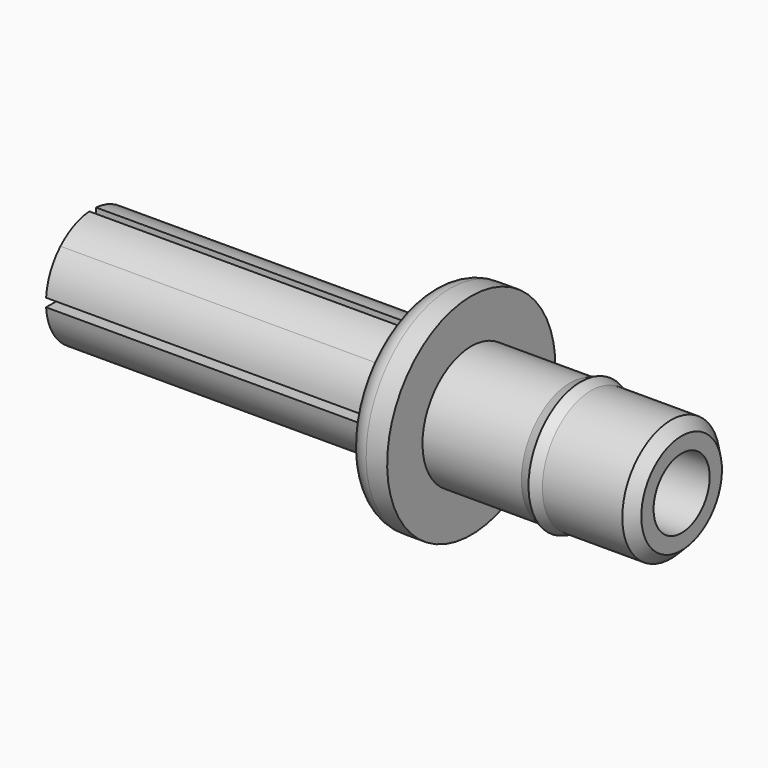
from build123d import *

# Parameters (mm, degrees)
F3_DEPTH = 15
F4_DEPTH = 15
F5_DEPTH = 15
F7_R     = 1


# Not quite as in the source:
# - after a boolean that leaves OpenCascade's solid faulty, fix() repairs it
# - a feature of the source that left no trace in its solid (it failed there, or was rolled back) is left out


with BuildPart() as f1:
    # F0 (on Front) → F1 (revolve)
    with BuildSketch(Plane.XZ):
        Polygon((2.7639019594, 2.7772041211), (2.7639019594, 1.666), (15.7639019594, 1.666), (15.7639019594, 2.3962433916), (15.2639019594, 2.9), (11.4639019594, 2.9), (10.9639019594, 3.1), (10.4639019594, 2.9), (5.7639019594, 2.9), (5.7639019594, 5), (3.7639019594, 5), (3.7639019594, 2.7772041211), align=None)
    revolve(axis=Axis((8.0730360566, 0, 0), (1, 0, 0)))

    # F2 (on face) → F3 (join)
    with BuildSketch(Plane(origin=(2.7639019594, 0, 0), x_dir=(0, -1, 0), z_dir=(-1, 0, 0))):
        with BuildLine():
            ThreePointArc((-1.1878670343, 1.1681300907), (-0.7352206258, 1.4949938566), (-0.2, 1.6539516317))
            Line((-0.2, 1.6539516317), (-0.2, 2.7699932726))
            ThreePointArc((-0.2, 2.7699932726), (-1.249471885, 2.4802586032), (-2.1069209339, 1.8093498579))
            ThreePointArc((-2.1069209339, 1.8093498579), (-2.5677957056, 1.0579640563), (-2.7699932726, 0.2))
            Line((-2.7699932726, 0.2), (-1.6539516317, 0.2))
            ThreePointArc((-1.6539516317, 0.2), (-1.5011003633, 0.7226712249), (-1.1878670343, 1.1681300907))
        make_face()
    extrude(amount=F3_DEPTH)

    # F2 (on face) → F4 (join)
    with BuildSketch(Plane(origin=(2.7639019594, 0, 0), x_dir=(0, -1, 0), z_dir=(-1, 0, 0))):
        with BuildLine():
            Line((0.2, 2.7699932726), (0.2, 1.6539516317))
            ThreePointArc((0.2, 1.6539516317), (0.75564146, 1.4847767455), (1.2194377654, 1.1351332681))
            ThreePointArc((1.2194377654, 1.1351332681), (1.5108640621, 0.7020297614), (1.6539516317, 0.2))
            Line((1.6539516317, 0.2), (2.7699932726, 0.2))
            ThreePointArc((2.7699932726, 0.2), (2.5121240066, 1.1841012226), (1.917164961, 2.0093136247))
            ThreePointArc((1.917164961, 2.0093136247), (1.1248356545, 2.5392139493), (0.2, 2.7699932726))
        make_face()
    extrude(amount=F4_DEPTH)

    # F2 (on face) → F5 (join)
    with BuildSketch(Plane(origin=(2.7639019594, 0, 0), x_dir=(0, -1, 0), z_dir=(-1, 0, 0))):
        with BuildLine():
            ThreePointArc((-1.1878670343, 1.1681300907), (-0.7352206258, 1.4949938566), (-0.2, 1.6539516317))
            Line((-0.2, 1.6539516317), (-0.2, 2.7699932726))
            ThreePointArc((-0.2, 2.7699932726), (-1.249471885, 2.4802586032), (-2.1069209339, 1.8093498579))
            ThreePointArc((-2.1069209339, 1.8093498579), (-2.5677957056, 1.0579640563), (-2.7699932726, 0.2))
            Line((-2.7699932726, 0.2), (-1.6539516317, 0.2))
            ThreePointArc((-1.6539516317, 0.2), (-1.5011003633, 0.7226712249), (-1.1878670343, 1.1681300907))
        make_face()
        with BuildLine():
            Line((0.2, 2.7699932726), (0.2, 1.6539516317))
            ThreePointArc((0.2, 1.6539516317), (0.75564146, 1.4847767455), (1.2194377654, 1.1351332681))
            ThreePointArc((1.2194377654, 1.1351332681), (1.5108640621, 0.7020297614), (1.6539516317, 0.2))
            Line((1.6539516317, 0.2), (2.7699932726, 0.2))
            ThreePointArc((2.7699932726, 0.2), (2.5121240066, 1.1841012226), (1.917164961, 2.0093136247))
            ThreePointArc((1.917164961, 2.0093136247), (1.1248356545, 2.5392139493), (0.2, 2.7699932726))
        make_face()
        with BuildLine():
            ThreePointArc((-0.2, -1.6539516317), (-1.1780398975, -1.1780398975), (-1.6539516317, -0.2))
            Line((-1.6539516317, -0.2), (-2.7699932726, -0.2))
            ThreePointArc((-2.7699932726, -0.2), (-1.9637798667, -1.9637798667), (-0.2, -2.7699932726))
            Line((-0.2, -2.7699932726), (-0.2, -1.6539516317))
        make_face()
        with BuildLine():
            Line((2.7699932726, -0.2), (1.6539516317, -0.2))
            ThreePointArc((1.6539516317, -0.2), (1.1780398975, -1.1780398975), (0.2, -1.6539516317))
            Line((0.2, -1.6539516317), (0.2, -2.7699932726))
            ThreePointArc((0.2, -2.7699932726), (1.9637798667, -1.9637798667), (2.7699932726, -0.2))
        make_face()
    extrude(amount=F5_DEPTH)

    add(f1.part.fix(), mode=Mode.REPLACE)

    # F7
    f7_edges = [f1.edges().sort_by_distance(p)[0] for p in [
        (3.763902, 0, -5),
    ]]
    fillet(f7_edges, radius=F7_R)


solid = f1.part
